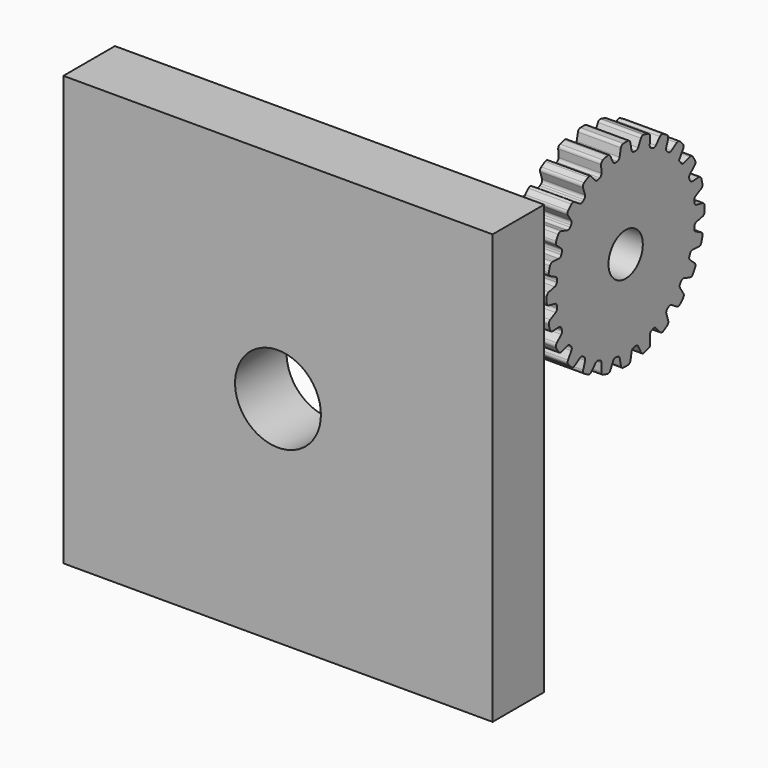
from build123d import *

# Parameters (mm, degrees)
F0_W         = 100
F0_H         = 100
F0_R         = 10
F1_DEPTH     = 15
F2_W         = 8
F2_H         = 18
F3_DEPTH     = 40
F4_R         = 5
F5_DEPTH     = 25
F6_R         = 23
F6_R_2       = 5
F7_DEPTH     = 10
F9_DEPTH     = 10
F10_T1_DEPTH = 10
F10_T3_DEPTH = 11.486760138
F10_T5_DEPTH = 12.957657443
F10_T7_DEPTH = 11.4788287215


# Not quite as in the source:
# - a fillet or chamfer that OpenCascade refuses, or shapes differently, is made with other operations: its cross-section is extruded or revolved along the edge and cut away or added


with BuildPart() as f1:
    # F0 (on Front) → F1 (new body)
    with BuildSketch(Plane.XZ):
        with Locations((50, 50)):
            Rectangle(F0_W, F0_H)
        with Locations((50, 50)):
            Circle(F0_R, mode=Mode.SUBTRACT)
    extrude(amount=F1_DEPTH)

    # F2 (on face) → F3 (join)
    with BuildSketch(Plane(origin=(0, 0, 0), x_dir=(-1, 0, 0), z_dir=(0, 1, 0))):
        with Locations((-81, 76)):
            Rectangle(F2_W, F2_H)
    extrude(amount=F3_DEPTH)

    # F4 (on face) → F5 (cut)
    with BuildSketch(Plane.YZ.offset(85)):
        with Locations((30, 76)):
            Circle(F4_R)
    extrude(amount=-F5_DEPTH, mode=Mode.SUBTRACT)

    # F6 (on face) → F7 (join)
    with BuildSketch(Plane.YZ.offset(85)):
        with Locations((30, 76)):
            Circle(F6_R)
        with Locations((30, 76)):
            Circle(F6_R_2, mode=Mode.SUBTRACT)
    extrude(amount=F7_DEPTH)

    # F8 (on face) → F9 (cut)
    with BuildSketch(Plane.YZ.offset(95)):
        with BuildLine():
            Line((33.3629795004, 95.8541875448), (34.7143450798, 98.5116625434))
            ThreePointArc((34.7143450798, 98.5116625434), (32.9790637867, 98.806253067), (31.2263361908, 98.9672832426))
            Line((31.2263361908, 98.9672832426), (31.8497418926, 96.0518540069))
            ThreePointArc((31.8497418926, 96.0518540069), (32.6150929247, 96.0198704372), (33.3629795004, 95.8541875448))
        make_face()
        with BuildLine():
            Line((38.3870306143, 94.3072693665), (40.3801546698, 96.5244339515))
            ThreePointArc((40.3801546698, 96.5244339515), (38.7802472909, 97.2581103937), (37.1289201158, 97.8672928819))
            Line((37.1289201158, 97.8672928819), (36.9765151727, 94.8898552199))
            ThreePointArc((36.9765151727, 94.8898552199), (37.7075095437, 94.6608740406), (38.3870306143, 94.3072693665))
        make_face()
        with BuildLine():
            Line((42.8395194521, 91.5127410351), (45.338573873, 93.1384991041))
            ThreePointArc((45.338573873, 93.1384991041), (43.9830714522, 94.2612626278), (42.5456799161, 95.2770826486))
            Line((42.5456799161, 95.2770826486), (41.6278504729, 92.4405440167))
            ThreePointArc((41.6278504729, 92.4405440167), (42.2746721246, 92.0301699168), (42.8395194521, 91.5127410351))
        make_face()
        with BuildLine():
            Line((46.4170162576, 87.6610450382), (49.251694615, 88.5846038654))
            ThreePointArc((49.251694615, 88.5846038654), (48.2329724023, 90.019939992), (47.1074723628, 91.3731710898))
            Line((47.1074723628, 91.3731710898), (45.4867669794, 88.8708369079))
            ThreePointArc((45.4867669794, 88.8708369079), (46.0053360851, 88.3070362042), (46.4170162576, 87.6610450382))
        make_face()
        with BuildLine():
            Line((48.8757205355, 83.0146680927), (51.8528441839, 83.1730886704))
            ThreePointArc((51.8528441839, 83.1730886704), (51.2403264145, 84.8231816147), (50.5034188394, 86.4216033265))
            Line((50.5034188394, 86.4216033265), (48.2902859093, 84.424003534))
            ThreePointArc((48.2902859093, 84.424003534), (48.6452628414, 83.7451983126), (48.8757205355, 83.0146680927))
        make_face()
        with BuildLine():
            Line((50.0480756525, 77.890253109), (52.9647585352, 77.2727393365))
            ThreePointArc((52.9647585352, 77.2727393365), (52.8001872828, 79.0251379915), (52.5020912056, 80.7598205191))
            Line((52.5020912056, 80.7598205191), (49.8473520806, 79.4030882405))
            ThreePointArc((49.8473520806, 79.4030882405), (50.0145457479, 78.6555379556), (50.0480756525, 77.890253109))
        make_face()
        with BuildLine():
            ThreePointArc((52.5116625434, 71.2856549202), (52.806253067, 73.0209362133), (52.9672832426, 74.7736638092))
            Line((52.9672832426, 74.7736638092), (50.0518540069, 74.1502581074))
            ThreePointArc((50.0518540069, 74.1502581074), (50.0198704372, 73.3849070753), (49.8541875448, 72.6370204996))
            Line((49.8541875448, 72.6370204996), (52.5116625434, 71.2856549202))
        make_face()
        with BuildLine():
            ThreePointArc((50.5244339515, 65.6198453302), (51.2581103937, 67.2197527091), (51.8672928819, 68.8710798842))
            Line((51.8672928819, 68.8710798842), (48.8898552199, 69.0234848273))
            ThreePointArc((48.8898552199, 69.0234848273), (48.6608740406, 68.2924904563), (48.3072693665, 67.6129693857))
            Line((48.3072693665, 67.6129693857), (50.5244339515, 65.6198453302))
        make_face()
        with BuildLine():
            ThreePointArc((47.1384991041, 60.661426127), (48.2612626278, 62.0169285478), (49.2770826486, 63.4543200839))
            Line((49.2770826486, 63.4543200839), (46.4405440167, 64.3721495271))
            ThreePointArc((46.4405440167, 64.3721495271), (46.0301699168, 63.7253278754), (45.5127410351, 63.1604805479))
            Line((45.5127410351, 63.1604805479), (47.1384991041, 60.661426127))
        make_face()
        with BuildLine():
            ThreePointArc((42.5846038654, 56.748305385), (44.019939992, 57.7670275977), (45.3731710898, 58.8925276372))
            Line((45.3731710898, 58.8925276372), (42.8708369079, 60.5132330206))
            ThreePointArc((42.8708369079, 60.5132330206), (42.3070362042, 59.9946639149), (41.6610450382, 59.5829837424))
            Line((41.6610450382, 59.5829837424), (42.5846038654, 56.748305385))
        make_face()
        with BuildLine():
            ThreePointArc((37.1730886704, 54.1471558161), (38.8231816147, 54.7596735855), (40.4216033265, 55.4965811606))
            Line((40.4216033265, 55.4965811606), (38.424003534, 57.7097140907))
            ThreePointArc((38.424003534, 57.7097140907), (37.7451983126, 57.3547371586), (37.0146680927, 57.1242794645))
            Line((37.0146680927, 57.1242794645), (37.1730886704, 54.1471558161))
        make_face()
        with BuildLine():
            ThreePointArc((31.2727393365, 53.0352414648), (33.0251379915, 53.1998127172), (34.7598205191, 53.4979087944))
            Line((34.7598205191, 53.4979087944), (33.4030882405, 56.1526479194))
            ThreePointArc((33.4030882405, 56.1526479194), (32.6555379556, 55.9854542521), (31.890253109, 55.9519243475))
            Line((31.890253109, 55.9519243475), (31.2727393365, 53.0352414648))
        make_face()
        with BuildLine():
            ThreePointArc((25.2856549202, 53.4883374566), (27.0209362133, 53.193746933), (28.7736638092, 53.0327167574))
            Line((28.7736638092, 53.0327167574), (28.1502581074, 55.9481459931))
            ThreePointArc((28.1502581074, 55.9481459931), (27.3849070753, 55.9801295628), (26.6370204996, 56.1458124552))
            Line((26.6370204996, 56.1458124552), (25.2856549202, 53.4883374566))
        make_face()
        with BuildLine():
            ThreePointArc((14.661426127, 58.8615008959), (16.0169285478, 57.7387373722), (17.4543200839, 56.7229173514))
            Line((17.4543200839, 56.7229173514), (18.3721495271, 59.5594559833))
            ThreePointArc((18.3721495271, 59.5594559833), (17.7253278754, 59.9698300832), (17.1604805479, 60.4872589649))
            Line((17.1604805479, 60.4872589649), (14.661426127, 58.8615008959))
        make_face()
        with BuildLine():
            ThreePointArc((10.748305385, 63.4153961346), (11.7670275977, 61.980060008), (12.8925276372, 60.6268289102))
            Line((12.8925276372, 60.6268289102), (14.5132330206, 63.1291630921))
            ThreePointArc((14.5132330206, 63.1291630921), (13.9946639149, 63.6929637958), (13.5829837424, 64.3389549618))
            Line((13.5829837424, 64.3389549618), (10.748305385, 63.4153961346))
        make_face()
        with BuildLine():
            ThreePointArc((8.1471558161, 68.8269113296), (8.7596735855, 67.1768183853), (9.4965811606, 65.5783966735))
            Line((9.4965811606, 65.5783966735), (11.7097140907, 67.575996466))
            ThreePointArc((11.7097140907, 67.575996466), (11.3547371586, 68.2548016874), (11.1242794645, 68.9853319073))
            Line((11.1242794645, 68.9853319073), (8.1471558161, 68.8269113296))
        make_face()
        with BuildLine():
            ThreePointArc((7.0352414648, 74.7272606635), (7.1998127172, 72.9748620085), (7.4979087944, 71.2401794809))
            Line((7.4979087944, 71.2401794809), (10.1526479194, 72.5969117595))
            ThreePointArc((10.1526479194, 72.5969117595), (9.9854542521, 73.3444620444), (9.9519243475, 74.109746891))
            Line((9.9519243475, 74.109746891), (7.0352414648, 74.7272606635))
        make_face()
        with BuildLine():
            Line((10.1458124552, 79.3629795004), (7.4883374566, 80.7143450798))
            ThreePointArc((7.4883374566, 80.7143450798), (7.193746933, 78.9790637867), (7.0327167574, 77.2263361908))
            Line((7.0327167574, 77.2263361908), (9.9481459931, 77.8497418926))
            ThreePointArc((9.9481459931, 77.8497418926), (9.9801295628, 78.6150929247), (10.1458124552, 79.3629795004))
        make_face()
        with BuildLine():
            Line((11.6927306335, 84.3870306143), (9.4755660485, 86.3801546698))
            ThreePointArc((9.4755660485, 86.3801546698), (8.7418896063, 84.7802472909), (8.1327071181, 83.1289201158))
            Line((8.1327071181, 83.1289201158), (11.1101447801, 82.9765151727))
            ThreePointArc((11.1101447801, 82.9765151727), (11.3391259594, 83.7075095437), (11.6927306335, 84.3870306143))
        make_face()
        with BuildLine():
            Line((14.4872589649, 88.8395194521), (12.8615008959, 91.338573873))
            ThreePointArc((12.8615008959, 91.338573873), (11.7387373722, 89.9830714522), (10.7229173514, 88.5456799161))
            Line((10.7229173514, 88.5456799161), (13.5594559833, 87.6278504729))
            ThreePointArc((13.5594559833, 87.6278504729), (13.9698300832, 88.2746721246), (14.4872589649, 88.8395194521))
        make_face()
        with BuildLine():
            Line((18.3389549618, 92.4170162576), (17.4153961346, 95.251694615))
            ThreePointArc((17.4153961346, 95.251694615), (15.980060008, 94.2329724023), (14.6268289102, 93.1074723628))
            Line((14.6268289102, 93.1074723628), (17.1291630921, 91.4867669794))
            ThreePointArc((17.1291630921, 91.4867669794), (17.6929637958, 92.0053360851), (18.3389549618, 92.4170162576))
        make_face()
        with BuildLine():
            Line((22.9853319073, 94.8757205355), (22.8269113296, 97.8528441839))
            ThreePointArc((22.8269113296, 97.8528441839), (21.1768183853, 97.2403264145), (19.5783966735, 96.5034188394))
            Line((19.5783966735, 96.5034188394), (21.575996466, 94.2902859093))
            ThreePointArc((21.575996466, 94.2902859093), (22.2548016874, 94.6452628414), (22.9853319073, 94.8757205355))
        make_face()
        with BuildLine():
            Line((28.109746891, 96.0480756525), (28.7272606635, 98.9647585352))
            ThreePointArc((28.7272606635, 98.9647585352), (26.9748620085, 98.8001872828), (25.2401794809, 98.5020912056))
            Line((25.2401794809, 98.5020912056), (26.5969117595, 95.8473520806))
            ThreePointArc((26.5969117595, 95.8473520806), (27.3444620444, 96.0145457479), (28.109746891, 96.0480756525))
        make_face()
        with BuildLine():
            ThreePointArc((19.6198453302, 55.4755660485), (21.2197527091, 54.7418896063), (22.8710798842, 54.1327071181))
            Line((22.8710798842, 54.1327071181), (23.0234848273, 57.1101447801))
            ThreePointArc((23.0234848273, 57.1101447801), (22.2924904563, 57.3391259594), (21.6129693857, 57.6927306335))
            Line((21.6129693857, 57.6927306335), (19.6198453302, 55.4755660485))
        make_face()
    extrude(amount=-F9_DEPTH, mode=Mode.SUBTRACT)

    # F10: fillet of radius 0.75 on 95 edges, made by hand

    # F10_s2 → F10_t1 (join)
    with BuildSketch(Plane.YZ.offset(85)):
        with BuildLine():
            ThreePointArc((22.0562087187, 94.5568894664), (21.5878875232, 94.4987026521), (21.1775238235, 94.731752178))
            Line((21.1775238235, 94.731752178), (21.575996466, 94.2902859093))
            ThreePointArc((21.575996466, 94.2902859093), (21.8118923496, 94.4311712706), (22.0562087187, 94.5568894664))
        make_face()
        with BuildLine():
            ThreePointArc((22.9537308497, 95.4695843974), (22.8292703064, 95.0143701393), (22.4575596482, 94.7236096981))
            ThreePointArc((22.4575596482, 94.7236096981), (22.719043621, 94.8079997742), (22.9853319073, 94.8757205355))
            Line((22.9853319073, 94.8757205355), (22.9537308497, 95.4695843974))
        make_face()
        with BuildLine():
            ThreePointArc((18.1547274064, 92.9824657435), (18.152325873, 92.5105497762), (17.868535288, 92.1334909592))
            ThreePointArc((17.868535288, 92.1334909592), (18.0992676516, 92.2826825453), (18.3389549618, 92.4170162576))
            Line((18.3389549618, 92.4170162576), (18.1547274064, 92.9824657435))
        make_face()
        with BuildLine():
            ThreePointArc((17.524010431, 91.8685743173), (17.0867067489, 91.6911597259), (16.6300081975, 91.810058341))
            Line((16.6300081975, 91.810058341), (17.1291630921, 91.4867669794))
            ThreePointArc((17.1291630921, 91.4867669794), (17.3205572037, 91.6839061358), (17.524010431, 91.8685743173))
        make_face()
        with BuildLine():
            ThreePointArc((27.1297632545, 95.9805832651), (26.662339861, 96.045589563), (26.3262766211, 96.3769080599))
            Line((26.3262766211, 96.3769080599), (26.5969117595, 95.8473520806))
            ThreePointArc((26.5969117595, 95.8473520806), (26.8612335005, 95.9223825423), (27.1297632545, 95.9805832651))
        make_face()
        with BuildLine():
            ThreePointArc((28.232925891, 96.6298830495), (27.9948881183, 96.2223926001), (27.5605888539, 96.0377453784))
            ThreePointArc((27.5605888539, 96.0377453784), (27.8350047353, 96.0515829002), (28.109746891, 96.0480756525))
            Line((28.109746891, 96.0480756525), (28.232925891, 96.6298830495))
        make_face()
        with BuildLine():
            ThreePointArc((32.3989196812, 96.0426333338), (31.9642482216, 96.2264026722), (31.7253875959, 96.6334113318))
            Line((31.7253875959, 96.6334113318), (31.8497418926, 96.0518540069))
            ThreePointArc((31.8497418926, 96.0518540069), (32.1244764012, 96.055916367), (32.3989196812, 96.0426333338))
        make_face()
        with BuildLine():
            ThreePointArc((33.6325441126, 96.3842892644), (33.2971509913, 96.0522924244), (32.8298598979, 95.986341825))
            ThreePointArc((32.8298598979, 95.986341825), (33.098506699, 95.9286837884), (33.3629795004, 95.8541875448))
            Line((33.3629795004, 95.8541875448), (33.6325441126, 96.3842892644))
        make_face()
        with BuildLine():
            ThreePointArc((14.1629597152, 89.3380201141), (14.282780852, 88.8815627308), (14.1062501998, 88.4439014732))
            ThreePointArc((14.1062501998, 88.4439014732), (14.2905069248, 88.6477274093), (14.4872589649, 88.8395194521))
            Line((14.4872589649, 88.8395194521), (14.1629597152, 89.3380201141))
        make_face()
        with BuildLine():
            ThreePointArc((13.8420302149, 88.0988420525), (13.4655455695, 87.8142901953), (12.9936354178, 87.8109351553))
            Line((12.9936354178, 87.8109351553), (13.5594559833, 87.6278504729))
            ThreePointArc((13.5594559833, 87.6278504729), (13.6933051306, 87.8678087167), (13.8420302149, 88.0988420525))
        make_face()
        with BuildLine():
            ThreePointArc((38.784610456, 94.7495398525), (38.3747184731, 94.5156616579), (37.9062806664, 94.5729021053))
            ThreePointArc((37.9062806664, 94.5729021053), (38.1508505518, 94.44767781), (38.3870306143, 94.3072693665))
            Line((38.3870306143, 94.3072693665), (38.784610456, 94.7495398525))
        make_face()
        with BuildLine():
            ThreePointArc((37.5045936961, 94.7388110627), (37.1322963119, 95.0288198649), (37.0069162573, 95.4837817199))
            Line((37.0069162573, 95.4837817199), (36.9765151727, 94.8898552199))
            ThreePointArc((36.9765151727, 94.8898552199), (37.242939746, 94.8226726353), (37.5045936961, 94.7388110627))
        make_face()
        with BuildLine():
            ThreePointArc((42.0988420525, 92.1579697851), (41.8142901953, 92.5344544305), (41.8109351553, 93.0063645822))
            Line((41.8109351553, 93.0063645822), (41.6278504729, 92.4405440167))
            ThreePointArc((41.6278504729, 92.4405440167), (41.8678087167, 92.3066948694), (42.0988420525, 92.1579697851))
        make_face()
        with BuildLine():
            ThreePointArc((43.3380201141, 91.8370402848), (42.8815627308, 91.717219148), (42.4439014732, 91.8937498002))
            ThreePointArc((42.4439014732, 91.8937498002), (42.6477274093, 91.7094930752), (42.8395194521, 91.5127410351))
            Line((42.8395194521, 91.5127410351), (43.3380201141, 91.8370402848))
        make_face()
        with BuildLine():
            ThreePointArc((13.0175342565, 64.1547274064), (13.4894502238, 64.152325873), (13.8665090408, 63.868535288))
            ThreePointArc((13.8665090408, 63.868535288), (13.7173174547, 64.0992676516), (13.5829837424, 64.3389549618))
            Line((13.5829837424, 64.3389549618), (13.0175342565, 64.1547274064))
        make_face()
        with BuildLine():
            ThreePointArc((14.1314256827, 63.524010431), (14.3088402741, 63.0867067489), (14.189941659, 62.6300081975))
            Line((14.189941659, 62.6300081975), (14.5132330206, 63.1291630921))
            ThreePointArc((14.5132330206, 63.1291630921), (14.3160938642, 63.3205572037), (14.1314256827, 63.524010431))
        make_face()
        with BuildLine():
            ThreePointArc((16.6619798859, 60.1629597152), (17.1184372692, 60.282780852), (17.5560985268, 60.1062501998))
            ThreePointArc((17.5560985268, 60.1062501998), (17.3522725907, 60.2905069248), (17.1604805479, 60.4872589649))
            Line((17.1604805479, 60.4872589649), (16.6619798859, 60.1629597152))
        make_face()
        with BuildLine():
            ThreePointArc((17.9011579475, 59.8420302149), (18.1857098047, 59.4655455695), (18.1890648447, 58.9936354178))
            Line((18.1890648447, 58.9936354178), (18.3721495271, 59.5594559833))
            ThreePointArc((18.3721495271, 59.5594559833), (18.1321912833, 59.6933051306), (17.9011579475, 59.8420302149))
        make_face()
        with BuildLine():
            ThreePointArc((21.215389544, 57.2504601475), (21.6252815269, 57.4843383421), (22.0937193336, 57.4270978947))
            ThreePointArc((22.0937193336, 57.4270978947), (21.8491494482, 57.55232219), (21.6129693857, 57.6927306335))
            Line((21.6129693857, 57.6927306335), (21.215389544, 57.2504601475))
        make_face()
        with BuildLine():
            ThreePointArc((22.4954063039, 57.2611889373), (22.8677036881, 56.9711801351), (22.9930837427, 56.5162182801))
            Line((22.9930837427, 56.5162182801), (23.0234848273, 57.1101447801))
            ThreePointArc((23.0234848273, 57.1101447801), (22.757060254, 57.1773273647), (22.4954063039, 57.2611889373))
        make_face()
        with BuildLine():
            ThreePointArc((26.3674558874, 55.6157107356), (26.7028490087, 55.9477075756), (27.1701401021, 56.013658175))
            ThreePointArc((27.1701401021, 56.013658175), (26.901493301, 56.0713162116), (26.6370204996, 56.1458124552))
            Line((26.6370204996, 56.1458124552), (26.3674558874, 55.6157107356))
        make_face()
        with BuildLine():
            ThreePointArc((27.6010803188, 55.9573666662), (28.0357517784, 55.7735973278), (28.2746124041, 55.3665886682))
            Line((28.2746124041, 55.3665886682), (28.1502581074, 55.9481459931))
            ThreePointArc((28.1502581074, 55.9481459931), (27.8755235988, 55.944083633), (27.6010803188, 55.9573666662))
        make_face()
        with BuildLine():
            ThreePointArc((31.767074109, 55.3701169505), (32.0051118817, 55.7776073999), (32.4394111461, 55.9622546216))
            ThreePointArc((32.4394111461, 55.9622546216), (32.1649952647, 55.9484170998), (31.890253109, 55.9519243475))
            Line((31.890253109, 55.9519243475), (31.767074109, 55.3701169505))
        make_face()
        with BuildLine():
            ThreePointArc((32.8702367455, 56.0194167349), (33.337660139, 55.954410437), (33.6737233789, 55.6230919401))
            Line((33.6737233789, 55.6230919401), (33.4030882405, 56.1526479194))
            ThreePointArc((33.4030882405, 56.1526479194), (33.1387664995, 56.0776174577), (32.8702367455, 56.0194167349))
        make_face()
        with BuildLine():
            ThreePointArc((37.0462691503, 56.5304156026), (37.1707296936, 56.9856298607), (37.5424403518, 57.2763903019))
            ThreePointArc((37.5424403518, 57.2763903019), (37.280956379, 57.1920002258), (37.0146680927, 57.1242794645))
            Line((37.0146680927, 57.1242794645), (37.0462691503, 56.5304156026))
        make_face()
        with BuildLine():
            ThreePointArc((37.9437912813, 57.4431105336), (38.4121124768, 57.5012973479), (38.8224761765, 57.268247822))
            Line((38.8224761765, 57.268247822), (38.424003534, 57.7097140907))
            ThreePointArc((38.424003534, 57.7097140907), (38.1881076504, 57.5688287294), (37.9437912813, 57.4431105336))
        make_face()
        with BuildLine():
            ThreePointArc((41.8452725936, 59.0175342565), (41.847674127, 59.4894502238), (42.131464712, 59.8665090408))
            ThreePointArc((42.131464712, 59.8665090408), (41.9007323484, 59.7173174547), (41.6610450382, 59.5829837424))
            Line((41.6610450382, 59.5829837424), (41.8452725936, 59.0175342565))
        make_face()
        with BuildLine():
            ThreePointArc((42.475989569, 60.1314256827), (42.9132932511, 60.3088402741), (43.3699918025, 60.189941659))
            Line((43.3699918025, 60.189941659), (42.8708369079, 60.5132330206))
            ThreePointArc((42.8708369079, 60.5132330206), (42.6794427963, 60.3160938642), (42.475989569, 60.1314256827))
        make_face()
        with BuildLine():
            ThreePointArc((45.8370402848, 62.6619798859), (45.717219148, 63.1184372692), (45.8937498002, 63.5560985268))
            ThreePointArc((45.8937498002, 63.5560985268), (45.7094930752, 63.3522725907), (45.5127410351, 63.1604805479))
            Line((45.5127410351, 63.1604805479), (45.8370402848, 62.6619798859))
        make_face()
        with BuildLine():
            ThreePointArc((46.1579697851, 63.9011579475), (46.5344544305, 64.1857098047), (47.0063645822, 64.1890648447))
            Line((47.0063645822, 64.1890648447), (46.4405440167, 64.3721495271))
            ThreePointArc((46.4405440167, 64.3721495271), (46.3066948694, 64.1321912833), (46.1579697851, 63.9011579475))
        make_face()
        with BuildLine():
            ThreePointArc((48.7495398525, 67.215389544), (48.5156616579, 67.6252815269), (48.5729021053, 68.0937193336))
            ThreePointArc((48.5729021053, 68.0937193336), (48.44767781, 67.8491494482), (48.3072693665, 67.6129693857))
            Line((48.3072693665, 67.6129693857), (48.7495398525, 67.215389544))
        make_face()
        with BuildLine():
            ThreePointArc((48.7388110627, 68.4954063039), (49.0288198649, 68.8677036881), (49.4837817199, 68.9930837427))
            Line((49.4837817199, 68.9930837427), (48.8898552199, 69.0234848273))
            ThreePointArc((48.8898552199, 69.0234848273), (48.8226726353, 68.757060254), (48.7388110627, 68.4954063039))
        make_face()
        with BuildLine():
            ThreePointArc((50.3842892644, 72.3674558874), (50.0522924244, 72.7028490087), (49.986341825, 73.1701401021))
            ThreePointArc((49.986341825, 73.1701401021), (49.9286837884, 72.901493301), (49.8541875448, 72.6370204996))
            Line((49.8541875448, 72.6370204996), (50.3842892644, 72.3674558874))
        make_face()
        with BuildLine():
            ThreePointArc((50.0426333338, 73.6010803188), (50.2264026722, 74.0357517784), (50.6334113318, 74.2746124041))
            Line((50.6334113318, 74.2746124041), (50.0518540069, 74.1502581074))
            ThreePointArc((50.0518540069, 74.1502581074), (50.055916367, 73.8755235988), (50.0426333338, 73.6010803188))
        make_face()
        with BuildLine():
            ThreePointArc((50.6298830495, 77.767074109), (50.2223926001, 78.0051118817), (50.0377453784, 78.4394111461))
            ThreePointArc((50.0377453784, 78.4394111461), (50.0515829002, 78.1649952647), (50.0480756525, 77.890253109))
            Line((50.0480756525, 77.890253109), (50.6298830495, 77.767074109))
        make_face()
        with BuildLine():
            ThreePointArc((49.9805832651, 78.8702367455), (50.045589563, 79.337660139), (50.3769080599, 79.6737233789))
            Line((50.3769080599, 79.6737233789), (49.8473520806, 79.4030882405))
            ThreePointArc((49.8473520806, 79.4030882405), (49.9223825423, 79.1387664995), (49.9805832651, 78.8702367455))
        make_face()
        with BuildLine():
            ThreePointArc((49.4695843974, 83.0462691503), (49.0143701393, 83.1707296936), (48.7236096981, 83.5424403518))
            ThreePointArc((48.7236096981, 83.5424403518), (48.8079997742, 83.280956379), (48.8757205355, 83.0146680927))
            Line((48.8757205355, 83.0146680927), (49.4695843974, 83.0462691503))
        make_face()
        with BuildLine():
            ThreePointArc((48.5568894664, 83.9437912813), (48.4987026521, 84.4121124768), (48.731752178, 84.8224761765))
            Line((48.731752178, 84.8224761765), (48.2902859093, 84.424003534))
            ThreePointArc((48.2902859093, 84.424003534), (48.4311712706, 84.1881076504), (48.5568894664, 83.9437912813))
        make_face()
        with BuildLine():
            ThreePointArc((46.9824657435, 87.8452725936), (46.5105497762, 87.847674127), (46.1334909592, 88.131464712))
            ThreePointArc((46.1334909592, 88.131464712), (46.2826825453, 87.9007323484), (46.4170162576, 87.6610450382))
            Line((46.4170162576, 87.6610450382), (46.9824657435, 87.8452725936))
        make_face()
    extrude(amount=F10_T1_DEPTH)

    # F10_s4 → F10_t3 (join)
    with BuildSketch(Plane.YZ.offset(83.513239862)):
        with BuildLine():
            ThreePointArc((11.4270978947, 83.9062806664), (11.4843383421, 84.3747184731), (11.2504601475, 84.784610456))
            Line((11.2504601475, 84.784610456), (11.6927306335, 84.3870306143))
            ThreePointArc((11.6927306335, 84.3870306143), (11.55232219, 84.1508505518), (11.4270978947, 83.9062806664))
        make_face()
        with BuildLine():
            ThreePointArc((11.2611889373, 83.5045936961), (10.9711801351, 83.1322963119), (10.5162182801, 83.0069162573))
            Line((10.5162182801, 83.0069162573), (11.1101447801, 82.9765151727))
            ThreePointArc((11.1101447801, 82.9765151727), (11.1773273647, 83.242939746), (11.2611889373, 83.5045936961))
        make_face()
        with BuildLine():
            ThreePointArc((9.6157107356, 79.6325441126), (9.9477075756, 79.2971509913), (10.013658175, 78.8298598979))
            ThreePointArc((10.013658175, 78.8298598979), (10.0713162116, 79.098506699), (10.1458124552, 79.3629795004))
            Line((10.1458124552, 79.3629795004), (9.6157107356, 79.6325441126))
        make_face()
        with BuildLine():
            ThreePointArc((9.9573666662, 78.3989196812), (9.7735973278, 77.9642482216), (9.3665886682, 77.7253875959))
            Line((9.3665886682, 77.7253875959), (9.9481459931, 77.8497418926))
            ThreePointArc((9.9481459931, 77.8497418926), (9.944083633, 78.1244764012), (9.9573666662, 78.3989196812))
        make_face()
        with BuildLine():
            ThreePointArc((9.3701169505, 74.232925891), (9.7776073999, 73.9948881183), (9.9622546216, 73.5605888539))
            ThreePointArc((9.9622546216, 73.5605888539), (9.9484170998, 73.8350047353), (9.9519243475, 74.109746891))
            Line((9.9519243475, 74.109746891), (9.3701169505, 74.232925891))
        make_face()
        with BuildLine():
            ThreePointArc((10.0194167349, 73.1297632545), (9.954410437, 72.662339861), (9.6230919401, 72.3262766211))
            Line((9.6230919401, 72.3262766211), (10.1526479194, 72.5969117595))
            ThreePointArc((10.1526479194, 72.5969117595), (10.0776174577, 72.8612335005), (10.0194167349, 73.1297632545))
        make_face()
        with BuildLine():
            ThreePointArc((10.5304156026, 68.9537308497), (10.9856298607, 68.8292703064), (11.2763903019, 68.4575596482))
            ThreePointArc((11.2763903019, 68.4575596482), (11.1920002258, 68.719043621), (11.1242794645, 68.9853319073))
            Line((11.1242794645, 68.9853319073), (10.5304156026, 68.9537308497))
        make_face()
        with BuildLine():
            ThreePointArc((11.4431105336, 68.0562087187), (11.5012973479, 67.5878875232), (11.268247822, 67.1775238235))
            Line((11.268247822, 67.1775238235), (11.7097140907, 67.575996466))
            ThreePointArc((11.7097140907, 67.575996466), (11.5688287294, 67.8118923496), (11.4431105336, 68.0562087187))
        make_face()
    extrude(amount=F10_T3_DEPTH)

    # F10_s6 → F10_t5 (cut)
    with BuildSketch(Plane.YZ.offset(83.5211712785)):
        with BuildLine():
            ThreePointArc((10.4066601529, 88.0457890416), (10.7860654643, 88.3566645273), (11.2764672636, 88.366565695))
            Line((11.2764672636, 88.366565695), (10.7229173514, 88.5456799161))
            ThreePointArc((10.7229173514, 88.5456799161), (10.563181614, 88.2967512388), (10.4066601529, 88.0457890416))
        make_face()
        with BuildLine():
            ThreePointArc((14.1919666356, 92.7064682429), (14.6389045209, 92.9085535829), (15.1151588949, 92.7911920511))
            Line((15.1151588949, 92.7911920511), (14.6268289102, 93.1074723628))
            ThreePointArc((14.6268289102, 93.1074723628), (14.4081085535, 92.9083683755), (14.1919666356, 92.7064682429))
        make_face()
        with BuildLine():
            ThreePointArc((13.1787672381, 90.850883933), (13.0604436687, 91.3269002046), (13.2616255532, 91.7742454932))
            ThreePointArc((13.2616255532, 91.7742454932), (13.0601625499, 91.5576960751), (12.8615008959, 91.338573873))
            Line((12.8615008959, 91.338573873), (13.1787672381, 90.850883933))
        make_face()
        with BuildLine():
            ThreePointArc((17.5956284438, 94.698507735), (17.604538729, 95.1889285387), (17.9146469875, 95.568961203))
            ThreePointArc((17.9146469875, 95.568961203), (17.6640015559, 95.4119329895), (17.4153961346, 95.251694615))
            Line((17.4153961346, 95.251694615), (17.5956284438, 94.698507735))
        make_face()
        with BuildLine():
            ThreePointArc((19.0545644682, 96.2286292422), (19.538576849, 96.3081526545), (19.9682278492, 96.0715264176))
            Line((19.9682278492, 96.0715264176), (19.5783966735, 96.5034188394))
            ThreePointArc((19.5783966735, 96.5034188394), (19.3155971283, 96.3677081498), (19.0545644682, 96.2286292422))
        make_face()
        with BuildLine():
            ThreePointArc((24.6630756441, 98.3722425881), (25.1511778766, 98.3237846836), (25.5049454972, 97.9840194286))
            Line((25.5049454972, 97.9840194286), (25.2401794809, 98.5020912056))
            ThreePointArc((25.2401794809, 98.5020912056), (24.951210102, 98.439022273), (24.6630756441, 98.3722425881))
        make_face()
        with BuildLine():
            ThreePointArc((28.6067529818, 98.3955684894), (28.8596799171, 98.8158302214), (29.318257879, 98.9898940337))
            ThreePointArc((29.318257879, 98.9898940337), (29.0226784612, 98.9792263275), (28.7272606635, 98.9647585352))
            Line((28.7272606635, 98.9647585352), (28.6067529818, 98.3955684894))
        make_face()
        with BuildLine():
            ThreePointArc((30.6352893951, 98.9912245734), (31.0942181188, 98.8180876782), (31.3479936812, 98.3983378458))
            Line((31.3479936812, 98.3983378458), (31.2263361908, 98.9672832426))
            ThreePointArc((31.2263361908, 98.9672832426), (30.9308897638, 98.9811541104), (30.6352893951, 98.9912245734))
        make_face()
        with BuildLine():
            ThreePointArc((34.4506263737, 97.9930568612), (34.8037067728, 98.333536214), (35.2917100992, 98.3829802356))
            ThreePointArc((35.2917100992, 98.3829802356), (35.0034413003, 98.4491776053), (34.7143450798, 98.5116625434))
            Line((34.7143450798, 98.5116625434), (34.4506263737, 97.9930568612))
        make_face()
        with BuildLine():
            ThreePointArc((22.8578270717, 97.2718591355), (22.9933639905, 97.7432631041), (23.3912652576, 98.030084546))
            ThreePointArc((23.3912652576, 98.030084546), (23.1085184698, 97.9432787504), (22.8269113296, 97.8528441839))
            Line((22.8269113296, 97.8528441839), (22.8578270717, 97.2718591355))
        make_face()
        with BuildLine():
            ThreePointArc((39.9911969332, 96.0917547532), (40.4203689504, 96.3292486216), (40.9045410212, 96.250703324))
            ThreePointArc((40.9045410212, 96.250703324), (40.6432278834, 96.3892545283), (40.3801546698, 96.5244339515))
            Line((40.3801546698, 96.5244339515), (39.9911969332, 96.0917547532))
        make_face()
        with BuildLine():
            ThreePointArc((36.5642092237, 98.0433925989), (36.9626892045, 97.7573757063), (37.0991783235, 97.2862465538))
            Line((37.0991783235, 97.2862465538), (37.1289201158, 97.8672928819))
            ThreePointArc((37.1289201158, 97.8672928819), (36.8471308265, 97.9571582734), (36.5642092237, 98.0433925989))
        make_face()
        with BuildLine():
            ThreePointArc((42.0457890416, 95.5933398471), (42.3566645273, 95.2139345357), (42.366565695, 94.7235327364))
            Line((42.366565695, 94.7235327364), (42.5456799161, 95.2770826486))
            ThreePointArc((42.5456799161, 95.2770826486), (42.2967512388, 95.436818386), (42.0457890416, 95.5933398471))
        make_face()
        with BuildLine():
            ThreePointArc((44.850883933, 92.8212327619), (45.3269002046, 92.9395563313), (45.7742454932, 92.7383744468))
            ThreePointArc((45.7742454932, 92.7383744468), (45.5576960751, 92.9398374501), (45.338573873, 93.1384991041))
            Line((45.338573873, 93.1384991041), (44.850883933, 92.8212327619))
        make_face()
        with BuildLine():
            ThreePointArc((9.9082452468, 85.9911969332), (9.6707513784, 86.4203689504), (9.749296676, 86.9045410212))
            ThreePointArc((9.749296676, 86.9045410212), (9.6107454717, 86.6432278834), (9.4755660485, 86.3801546698))
            Line((9.4755660485, 86.3801546698), (9.9082452468, 85.9911969332))
        make_face()
        with BuildLine():
            ThreePointArc((9.9284735824, 65.9682278492), (9.6918473455, 65.538576849), (9.7713707578, 65.0545644682))
            ThreePointArc((9.7713707578, 65.0545644682), (9.6322918502, 65.3155971283), (9.4965811606, 65.5783966735))
            Line((9.4965811606, 65.5783966735), (9.9284735824, 65.9682278492))
        make_face()
        with BuildLine():
            ThreePointArc((11.301492265, 63.5956284438), (10.8110714613, 63.604538729), (10.431038797, 63.9146469875))
            ThreePointArc((10.431038797, 63.9146469875), (10.5880670105, 63.6640015559), (10.748305385, 63.4153961346))
            Line((10.748305385, 63.4153961346), (11.301492265, 63.5956284438))
        make_face()
        with BuildLine():
            ThreePointArc((13.2935317571, 60.1919666356), (13.0914464171, 60.6389045209), (13.2088079489, 61.1151588949))
            Line((13.2088079489, 61.1151588949), (12.8925276372, 60.6268289102))
            ThreePointArc((12.8925276372, 60.6268289102), (13.0916316245, 60.4081085535), (13.2935317571, 60.1919666356))
        make_face()
        with BuildLine():
            ThreePointArc((15.149116067, 59.1787672381), (14.6730997954, 59.0604436687), (14.2257545068, 59.2616255532))
            ThreePointArc((14.2257545068, 59.2616255532), (14.4423039249, 59.0601625499), (14.661426127, 58.8615008959))
            Line((14.661426127, 58.8615008959), (15.149116067, 59.1787672381))
        make_face()
        with BuildLine():
            ThreePointArc((17.9542109584, 56.4066601529), (17.6433354727, 56.7860654643), (17.633434305, 57.2764672636))
            Line((17.633434305, 57.2764672636), (17.4543200839, 56.7229173514))
            ThreePointArc((17.4543200839, 56.7229173514), (17.7032487612, 56.563181614), (17.9542109584, 56.4066601529))
        make_face()
        with BuildLine():
            ThreePointArc((20.0088030668, 55.9082452468), (19.5796310496, 55.6707513784), (19.0954589788, 55.749296676))
            ThreePointArc((19.0954589788, 55.749296676), (19.3567721166, 55.6107454717), (19.6198453302, 55.4755660485))
            Line((19.6198453302, 55.4755660485), (20.0088030668, 55.9082452468))
        make_face()
        with BuildLine():
            ThreePointArc((23.4357907763, 53.9566074011), (23.0373107955, 54.2426242937), (22.9008216765, 54.7137534462))
            Line((22.9008216765, 54.7137534462), (22.8710798842, 54.1327071181))
            ThreePointArc((22.8710798842, 54.1327071181), (23.1528691735, 54.0428417266), (23.4357907763, 53.9566074011))
        make_face()
        with BuildLine():
            ThreePointArc((25.5493736263, 54.0069431388), (25.1962932272, 53.666463786), (24.7082899008, 53.6170197644))
            ThreePointArc((24.7082899008, 53.6170197644), (24.9965586997, 53.5508223947), (25.2856549202, 53.4883374566))
            Line((25.2856549202, 53.4883374566), (25.5493736263, 54.0069431388))
        make_face()
        with BuildLine():
            ThreePointArc((29.3647106049, 53.0087754266), (28.9057818812, 53.1819123218), (28.6520063188, 53.6016621542))
            Line((28.6520063188, 53.6016621542), (28.7736638092, 53.0327167574))
            ThreePointArc((28.7736638092, 53.0327167574), (29.0691102362, 53.0188458896), (29.3647106049, 53.0087754266))
        make_face()
        with BuildLine():
            ThreePointArc((31.3932470182, 53.6044315106), (31.1403200829, 53.1841697786), (30.681742121, 53.0101059663))
            ThreePointArc((30.681742121, 53.0101059663), (30.9773215388, 53.0207736725), (31.2727393365, 53.0352414648))
            Line((31.2727393365, 53.0352414648), (31.3932470182, 53.6044315106))
        make_face()
        with BuildLine():
            ThreePointArc((35.3369243559, 53.6277574119), (34.8488221234, 53.6762153164), (34.4950545028, 54.0159805714))
            Line((34.4950545028, 54.0159805714), (34.7598205191, 53.4979087944))
            ThreePointArc((34.7598205191, 53.4979087944), (35.048789898, 53.560977727), (35.3369243559, 53.6277574119))
        make_face()
        with BuildLine():
            ThreePointArc((37.1421729283, 54.7281408645), (37.0066360095, 54.2567368959), (36.6087347424, 53.969915454))
            ThreePointArc((36.6087347424, 53.969915454), (36.8914815302, 54.0567212496), (37.1730886704, 54.1471558161))
            Line((37.1730886704, 54.1471558161), (37.1421729283, 54.7281408645))
        make_face()
        with BuildLine():
            ThreePointArc((40.9454355318, 55.7713707578), (40.461423151, 55.6918473455), (40.0317721508, 55.9284735824))
            Line((40.0317721508, 55.9284735824), (40.4216033265, 55.4965811606))
            ThreePointArc((40.4216033265, 55.4965811606), (40.6844028717, 55.6322918502), (40.9454355318, 55.7713707578))
        make_face()
        with BuildLine():
            ThreePointArc((42.4043715562, 57.301492265), (42.395461271, 56.8110714613), (42.0853530125, 56.431038797))
            ThreePointArc((42.0853530125, 56.431038797), (42.3359984441, 56.5880670105), (42.5846038654, 56.748305385))
            Line((42.5846038654, 56.748305385), (42.4043715562, 57.301492265))
        make_face()
        with BuildLine():
            ThreePointArc((45.8080333644, 59.2935317571), (45.3610954791, 59.0914464171), (44.8848411051, 59.2088079489))
            Line((44.8848411051, 59.2088079489), (45.3731710898, 58.8925276372))
            ThreePointArc((45.3731710898, 58.8925276372), (45.5918914465, 59.0916316245), (45.8080333644, 59.2935317571))
        make_face()
        with BuildLine():
            ThreePointArc((46.8212327619, 61.149116067), (46.9395563313, 60.6730997954), (46.7383744468, 60.2257545068))
            ThreePointArc((46.7383744468, 60.2257545068), (46.9398374501, 60.4423039249), (47.1384991041, 60.661426127))
            Line((47.1384991041, 60.661426127), (46.8212327619, 61.149116067))
        make_face()
        with BuildLine():
            ThreePointArc((49.5933398471, 63.9542109584), (49.2139345357, 63.6433354727), (48.7235327364, 63.633434305))
            Line((48.7235327364, 63.633434305), (49.2770826486, 63.4543200839))
            ThreePointArc((49.2770826486, 63.4543200839), (49.436818386, 63.7032487612), (49.5933398471, 63.9542109584))
        make_face()
        with BuildLine():
            ThreePointArc((50.0917547532, 66.0088030668), (50.3292486216, 65.5796310496), (50.250703324, 65.0954589788))
            ThreePointArc((50.250703324, 65.0954589788), (50.3892545283, 65.3567721166), (50.5244339515, 65.6198453302))
            Line((50.5244339515, 65.6198453302), (50.0917547532, 66.0088030668))
        make_face()
        with BuildLine():
            ThreePointArc((52.0433925989, 69.4357907763), (51.7573757063, 69.0373107955), (51.2862465538, 68.9008216765))
            Line((51.2862465538, 68.9008216765), (51.8672928819, 68.8710798842))
            ThreePointArc((51.8672928819, 68.8710798842), (51.9571582734, 69.1528691735), (52.0433925989, 69.4357907763))
        make_face()
        with BuildLine():
            ThreePointArc((51.9930568612, 71.5493736263), (52.333536214, 71.1962932272), (52.3829802356, 70.7082899008))
            ThreePointArc((52.3829802356, 70.7082899008), (52.4491776053, 70.9965586997), (52.5116625434, 71.2856549202))
            Line((52.5116625434, 71.2856549202), (51.9930568612, 71.5493736263))
        make_face()
        with BuildLine():
            ThreePointArc((52.9912245734, 75.3647106049), (52.8180876782, 74.9057818812), (52.3983378458, 74.6520063188))
            Line((52.3983378458, 74.6520063188), (52.9672832426, 74.7736638092))
            ThreePointArc((52.9672832426, 74.7736638092), (52.9811541104, 75.0691102362), (52.9912245734, 75.3647106049))
        make_face()
        with BuildLine():
            ThreePointArc((52.3955684894, 77.3932470182), (52.8158302214, 77.1403200829), (52.9898940337, 76.681742121))
            ThreePointArc((52.9898940337, 76.681742121), (52.9792263275, 76.9773215388), (52.9647585352, 77.2727393365))
            Line((52.9647585352, 77.2727393365), (52.3955684894, 77.3932470182))
        make_face()
        with BuildLine():
            ThreePointArc((52.3722425881, 81.3369243559), (52.3237846836, 80.8488221234), (51.9840194286, 80.4950545028))
            Line((51.9840194286, 80.4950545028), (52.5020912056, 80.7598205191))
            ThreePointArc((52.5020912056, 80.7598205191), (52.439022273, 81.048789898), (52.3722425881, 81.3369243559))
        make_face()
        with BuildLine():
            ThreePointArc((51.2718591355, 83.1421729283), (51.7432631041, 83.0066360095), (52.030084546, 82.6087347424))
            ThreePointArc((52.030084546, 82.6087347424), (51.9432787504, 82.8914815302), (51.8528441839, 83.1730886704))
            Line((51.8528441839, 83.1730886704), (51.2718591355, 83.1421729283))
        make_face()
        with BuildLine():
            ThreePointArc((50.2286292422, 86.9454355318), (50.3081526545, 86.461423151), (50.0715264176, 86.0317721508))
            Line((50.0715264176, 86.0317721508), (50.5034188394, 86.4216033265))
            ThreePointArc((50.5034188394, 86.4216033265), (50.3677081498, 86.6844028717), (50.2286292422, 86.9454355318))
        make_face()
        with BuildLine():
            ThreePointArc((48.698507735, 88.4043715562), (49.1889285387, 88.395461271), (49.568961203, 88.0853530125))
            ThreePointArc((49.568961203, 88.0853530125), (49.4119329895, 88.3359984441), (49.251694615, 88.5846038654))
            Line((49.251694615, 88.5846038654), (48.698507735, 88.4043715562))
        make_face()
        with BuildLine():
            ThreePointArc((46.7064682429, 91.8080333644), (46.9085535829, 91.3610954791), (46.7911920511, 90.8848411051))
            Line((46.7911920511, 90.8848411051), (47.1074723628, 91.3731710898))
            ThreePointArc((47.1074723628, 91.3731710898), (46.9083683755, 91.5918914465), (46.7064682429, 91.8080333644))
        make_face()
    extrude(amount=F10_T5_DEPTH, mode=Mode.SUBTRACT)

    # F10_s8 → F10_t7 (cut)
    with BuildSketch(Plane.YZ.offset(85)):
        with BuildLine():
            ThreePointArc((7.9566074011, 82.5642092237), (8.2426242937, 82.9626892045), (8.7137534462, 83.0991783235))
            Line((8.7137534462, 83.0991783235), (8.1327071181, 83.1289201158))
            ThreePointArc((8.1327071181, 83.1289201158), (8.0428417266, 82.8471308265), (7.9566074011, 82.5642092237))
        make_face()
        with BuildLine():
            ThreePointArc((8.0069431388, 80.4506263737), (7.666463786, 80.8037067728), (7.6170197644, 81.2917100992))
            ThreePointArc((7.6170197644, 81.2917100992), (7.5508223947, 81.0034413003), (7.4883374566, 80.7143450798))
            Line((7.4883374566, 80.7143450798), (8.0069431388, 80.4506263737))
        make_face()
        with BuildLine():
            ThreePointArc((7.0087754266, 76.6352893951), (7.1819123218, 77.0942181188), (7.6016621542, 77.3479936812))
            Line((7.6016621542, 77.3479936812), (7.0327167574, 77.2263361908))
            ThreePointArc((7.0327167574, 77.2263361908), (7.0188458896, 76.9308897638), (7.0087754266, 76.6352893951))
        make_face()
        with BuildLine():
            ThreePointArc((7.6044315106, 74.6067529818), (7.1841697786, 74.8596799171), (7.0101059663, 75.318257879))
            ThreePointArc((7.0101059663, 75.318257879), (7.0207736725, 75.0226784612), (7.0352414648, 74.7272606635))
            Line((7.0352414648, 74.7272606635), (7.6044315106, 74.6067529818))
        make_face()
        with BuildLine():
            ThreePointArc((7.6277574119, 70.6630756441), (7.6762153164, 71.1511778766), (8.0159805714, 71.5049454972))
            Line((8.0159805714, 71.5049454972), (7.4979087944, 71.2401794809))
            ThreePointArc((7.4979087944, 71.2401794809), (7.560977727, 70.951210102), (7.6277574119, 70.6630756441))
        make_face()
        with BuildLine():
            ThreePointArc((8.7281408645, 68.8578270717), (8.2567368959, 68.9933639905), (7.969915454, 69.3912652576))
            ThreePointArc((7.969915454, 69.3912652576), (8.0567212496, 69.1085184698), (8.1471558161, 68.8269113296))
            Line((8.1471558161, 68.8269113296), (8.7281408645, 68.8578270717))
        make_face()
    extrude(amount=F10_T7_DEPTH, mode=Mode.SUBTRACT)


solid = f1.part
